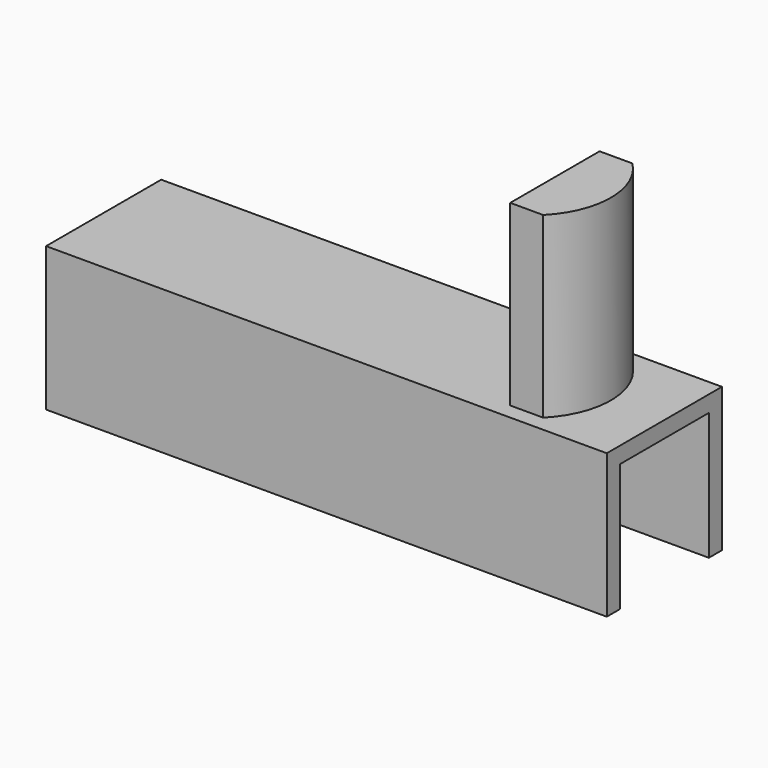
from build123d import *

# Parameters (mm, degrees)
F0_W     = 34.925
F0_H     = 8.9647058824
F1_DEPTH = 8.9647058824
F2_W     = 6.9327058824
F2_H     = 7.9487058824
F3_DEPTH = 34.926
F4_W     = 2.0463057544
F4_H     = 6.9543164351
F5_DEPTH = 11.1125


# Not quite as in the source:
# - a length typed as a fraction of an inch, garbled in the dataset ("3 / 203.2 mm" for 3/8 in), is restored


with BuildPart() as f1:
    # F0 (on Top) → F1 (new body)
    with BuildSketch(Plane.XY):
        with Locations((-7.0361781826, 4.5039634939)):
            Rectangle(F0_W, F0_H)
    extrude(amount=F1_DEPTH)

    # F2 (on face) → F3 (cut, through all)
    with BuildSketch(Plane.YZ.offset(10.4263218174)):
        with Locations((4.5039634939, 3.9743529412)):
            Rectangle(F2_W, F2_H)
    extrude(amount=-F3_DEPTH, mode=Mode.SUBTRACT)

    # F4 (on face) → F5 (join)
    with BuildSketch(Plane.XY.offset(8.9647058824)):
        with BuildLine():
            ThreePointArc((5.6638218174, 1.016), (7.1045145349, 4.4931582176), (5.6638218174, 7.9703164351))
            Line((5.6638218174, 7.9703164351), (5.6638218174, 1.016))
        make_face()
        with Locations((4.6406689402, 4.4931582176)):
            Rectangle(F4_W, F4_H)
    extrude(amount=F5_DEPTH)


solid = f1.part
